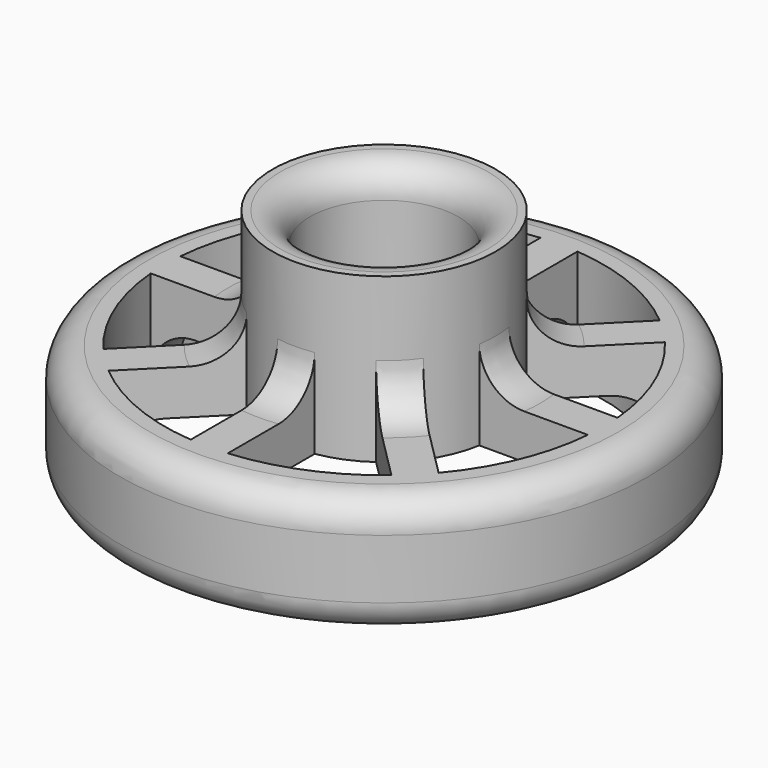
from build123d import *

# Parameters (mm, degrees)
F0_R     = 17.75
F0_R_2   = 14.75
F1_DEPTH = 8
F3_R     = 7.5
F3_R_2   = 5
F4_DEPTH = 11
F5_W     = 2.4922459852
F5_H     = 8.3065871149
F6_DEPTH = 3
F8_COUNT = 8
F9_R     = 3
F10_R    = 2


with BuildPart() as f1:
    # F0 (on Top) → F1 (new body)
    with BuildSketch(Plane.XY):
        Circle(F0_R)
        Circle(F0_R_2, mode=Mode.SUBTRACT)
    extrude(amount=F1_DEPTH)



with BuildPart() as f4:
    # F3 (on offset) → F4 (new body)
    with BuildSketch(Plane.XY.offset(5)):
        Circle(F3_R)
        Circle(F3_R_2, mode=Mode.SUBTRACT)
    extrude(amount=F4_DEPTH)


with BuildPart() as f1_1:
    add(f1.part)

    add(f4.part)  # F6 merges F4
    # F5 (on offset) → F6 (join)
    with BuildSketch(Plane.XY.offset(5)):
        with Locations((0, 11.1227082089)):
            Rectangle(F5_W, F5_H)
    extrude(amount=F6_DEPTH)

    # F8: F1 ×8 about axis
    f8_axis = Axis((0, 0, 7.9989284277), (0, 0, -1))


with BuildPart() as f1_2:
    add(f1_1.part)
    for i in range(1, F8_COUNT):
        add(f1_1.part.rotate(f8_axis, i * 360 / F8_COUNT))

    # F9
    f9_edges = [f1_2.edges().sort_by_distance(p)[0] for p in [
        (7.473893, 0.625238, 8),
        (7.473893, -0.625238, 8),
        (5.303301, -5.303301, 8),
        (0, -7.5, 8),
        (-5.303301, -5.303301, 8),
        (-7.5, 0, 8),
        (-5.303301, 5.303301, 8),
        (0, 7.5, 8),
        (5.303301, 5.303301, 8),
        (14.736811, 0.623619, 5),
        (10.429825, 10.429825, 5),
        (0, 14.75, 5),
        (-10.429825, 10.429825, 5),
        (-14.75, 0, 5),
        (-10.429825, -10.429825, 5),
        (0, -14.75, 5),
        (10.429825, -10.429825, 5),
        (14.736811, -0.623619, 5),
    ]]
    fillet(f9_edges, radius=F9_R)

    # F10
    f10_edges = [f1_2.edges().sort_by_distance(p)[0] for p in [
        (-17.75, 0, 8),
        (-17.75, 0, 0),
        (-5, 0, 16),
    ]]
    fillet(f10_edges, radius=F10_R)


solid = f1_2.part
